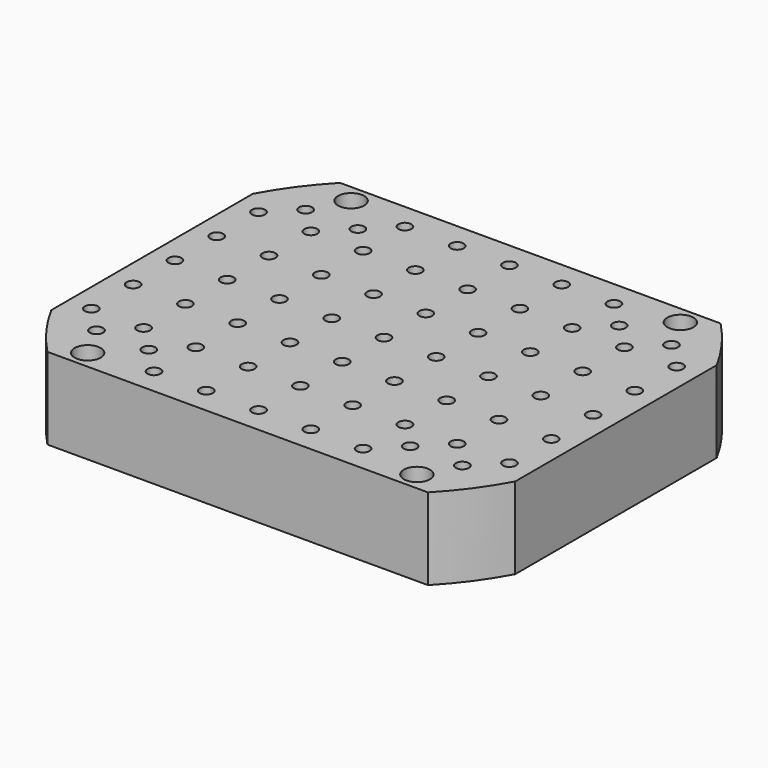
from build123d import *

# Parameters (mm, degrees)
F0_W      = 450.85
F0_H      = 355.6
F1_DEPTH  = 79.375
F3_DEPTH  = 79.376
F4_R      = 12.7
F4_R_2    = 8.5328125
F5_DEPTH  = 38.1
F6_DEPTH  = 79.376
F7_R      = 6.35
F8_DEPTH  = 79.376
F9_R      = 6.35
F10_DEPTH = 79.376


with BuildPart() as f1:
    # F0 (on Top) → F1 (new body)
    with BuildSketch(Plane.XY):
        with Locations((-225.425, -177.8)):
            Rectangle(F0_W, F0_H)
    extrude(amount=-F1_DEPTH)

    # F2 (on face) → F3 (cut, through all)
    with BuildSketch(Plane.XY):
        with BuildLine():
            ThreePointArc((-40.4927648434, 0), (-18.3889970697, -26.3111717299), (0, -55.3404516789))
            Line((0, -55.3404516789), (0, 0))
            Line((0, 0), (-40.4927648434, 0))
        make_face()
        with BuildLine():
            Line((0, -355.6), (0, -300.2595483211))
            ThreePointArc((0, -300.2595483211), (-18.3889970697, -329.2888282701), (-40.4927648434, -355.6))
            Line((-40.4927648434, -355.6), (0, -355.6))
        make_face()
        with BuildLine():
            ThreePointArc((-410.3572351566, -355.6), (-225.425, -434.34), (-40.4927648434, -355.6))
            Line((-40.4927648434, -355.6), (-410.3572351566, -355.6))
        make_face()
        with BuildLine():
            ThreePointArc((-450.85, -55.3404516789), (-432.4610029303, -26.3111717299), (-410.3572351566, 0))
            Line((-410.3572351566, 0), (-450.85, 0))
            Line((-450.85, 0), (-450.85, -55.3404516789))
        make_face()
        with BuildLine():
            Line((-450.85, -355.6), (-410.3572351566, -355.6))
            ThreePointArc((-410.3572351566, -355.6), (-432.4610029303, -329.2888282701), (-450.85, -300.2595483211))
            Line((-450.85, -300.2595483211), (-450.85, -355.6))
        make_face()
    extrude(amount=-F3_DEPTH, mode=Mode.SUBTRACT)

    # F4 (on face) → F5 (cut)
    with BuildSketch(Plane.XY):
        with Locations((-385.445, -337.82)):
            Circle(F4_R)
        with Locations((-385.445, -337.82)):
            Circle(F4_R_2, mode=Mode.SUBTRACT)
        with Locations((-65.405, -17.78)):
            Circle(F4_R)
        with Locations((-65.405, -17.78)):
            Circle(F4_R_2, mode=Mode.SUBTRACT)
        with Locations((-65.405, -337.82)):
            Circle(F4_R)
        with Locations((-65.405, -337.82)):
            Circle(F4_R_2, mode=Mode.SUBTRACT)
        with Locations((-385.445, -17.78)):
            Circle(F4_R)
        with Locations((-385.445, -17.78)):
            Circle(F4_R_2, mode=Mode.SUBTRACT)
    extrude(amount=-F5_DEPTH, mode=Mode.SUBTRACT)

    # F4 (on face) → F6 (cut, through all)
    with BuildSketch(Plane.XY):
        with Locations((-385.445, -337.82)):
            Circle(F4_R_2)
        with Locations((-65.405, -337.82)):
            Circle(F4_R_2)
        with Locations((-65.405, -17.78)):
            Circle(F4_R_2)
        with Locations((-385.445, -17.78)):
            Circle(F4_R_2)
    extrude(amount=-F6_DEPTH, mode=Mode.SUBTRACT)

    # F7 (on face) → F8 (cut, through all)
    with BuildSketch(Plane.XY):
        with Locations((-377.825, -76.2)):
            Circle(F7_R)
        with Locations((-428.625, -76.2)):
            Circle(F7_R)
        with Locations((-327.025, -25.4)):
            Circle(F7_R)
        with Locations((-276.225, -25.4)):
            Circle(F7_R)
        with Locations((-225.425, -25.4)):
            Circle(F7_R)
        with Locations((-174.625, -25.4)):
            Circle(F7_R)
        with Locations((-123.825, -25.4)):
            Circle(F7_R)
        with Locations((-73.025, -76.2)):
            Circle(F7_R)
        with Locations((-123.825, -127)):
            Circle(F7_R)
        with Locations((-73.025, -127)):
            Circle(F7_R)
        with Locations((-22.225, -127)):
            Circle(F7_R)
        with Locations((-22.225, -76.2)):
            Circle(F7_R)
        with Locations((-123.825, -76.2)):
            Circle(F7_R)
        with Locations((-174.625, -76.2)):
            Circle(F7_R)
        with Locations((-225.425, -76.2)):
            Circle(F7_R)
        with Locations((-276.225, -76.2)):
            Circle(F7_R)
        with Locations((-327.025, -76.2)):
            Circle(F7_R)
        with Locations((-428.625, -127)):
            Circle(F7_R)
        with Locations((-327.025, -127)):
            Circle(F7_R)
        with Locations((-276.225, -127)):
            Circle(F7_R)
        with Locations((-225.425, -127)):
            Circle(F7_R)
        with Locations((-174.625, -127)):
            Circle(F7_R)
        with Locations((-225.425, -177.8)):
            Circle(F7_R)
        with Locations((-276.225, -177.8)):
            Circle(F7_R)
        with Locations((-327.025, -177.8)):
            Circle(F7_R)
        with Locations((-377.825, -177.8)):
            Circle(F7_R)
        with Locations((-428.625, -177.8)):
            Circle(F7_R)
        with Locations((-174.625, -177.8)):
            Circle(F7_R)
        with Locations((-73.025, -177.8)):
            Circle(F7_R)
        with Locations((-123.825, -177.8)):
            Circle(F7_R)
        with Locations((-22.225, -177.8)):
            Circle(F7_R)
        with Locations((-22.225, -228.6)):
            Circle(F7_R)
        with Locations((-123.825, -228.6)):
            Circle(F7_R)
        with Locations((-174.625, -228.6)):
            Circle(F7_R)
        with Locations((-73.025, -228.6)):
            Circle(F7_R)
        with Locations((-225.425, -228.6)):
            Circle(F7_R)
        with Locations((-276.225, -228.6)):
            Circle(F7_R)
        with Locations((-327.025, -228.6)):
            Circle(F7_R)
        with Locations((-377.825, -127)):
            Circle(F7_R)
        with Locations((-377.825, -228.6)):
            Circle(F7_R)
        with Locations((-428.625, -228.6)):
            Circle(F7_R)
        with Locations((-327.025, -279.4)):
            Circle(F7_R)
        with Locations((-377.825, -279.4)):
            Circle(F7_R)
        with Locations((-428.625, -279.4)):
            Circle(F7_R)
        with Locations((-276.225, -279.4)):
            Circle(F7_R)
        with Locations((-225.425, -279.4)):
            Circle(F7_R)
        with Locations((-22.225, -279.4)):
            Circle(F7_R)
        with Locations((-123.825, -330.2)):
            Circle(F7_R)
        with Locations((-174.625, -330.2)):
            Circle(F7_R)
        with Locations((-225.425, -330.2)):
            Circle(F7_R)
        with Locations((-174.625, -279.4)):
            Circle(F7_R)
        with Locations((-123.825, -279.4)):
            Circle(F7_R)
        with Locations((-73.025, -279.4)):
            Circle(F7_R)
        with Locations((-276.225, -330.2)):
            Circle(F7_R)
        with Locations((-327.025, -330.2)):
            Circle(F7_R)
    extrude(amount=-F8_DEPTH, mode=Mode.SUBTRACT)

    # F9 (on face) → F10 (cut, through all)
    with BuildSketch(Plane.XY):
        with Locations((-403.225, -304.8)):
            Circle(F9_R)
        with Locations((-352.425, -304.8)):
            Circle(F9_R)
        with Locations((-352.425, -50.8)):
            Circle(F9_R)
        with Locations((-403.225, -50.8)):
            Circle(F9_R)
        with Locations((-98.425, -50.8)):
            Circle(F9_R)
        with Locations((-47.625, -50.8)):
            Circle(F9_R)
        with Locations((-98.425, -304.8)):
            Circle(F9_R)
        with Locations((-47.625, -304.8)):
            Circle(F9_R)
    extrude(amount=-F10_DEPTH, mode=Mode.SUBTRACT)


solid = f1.part
